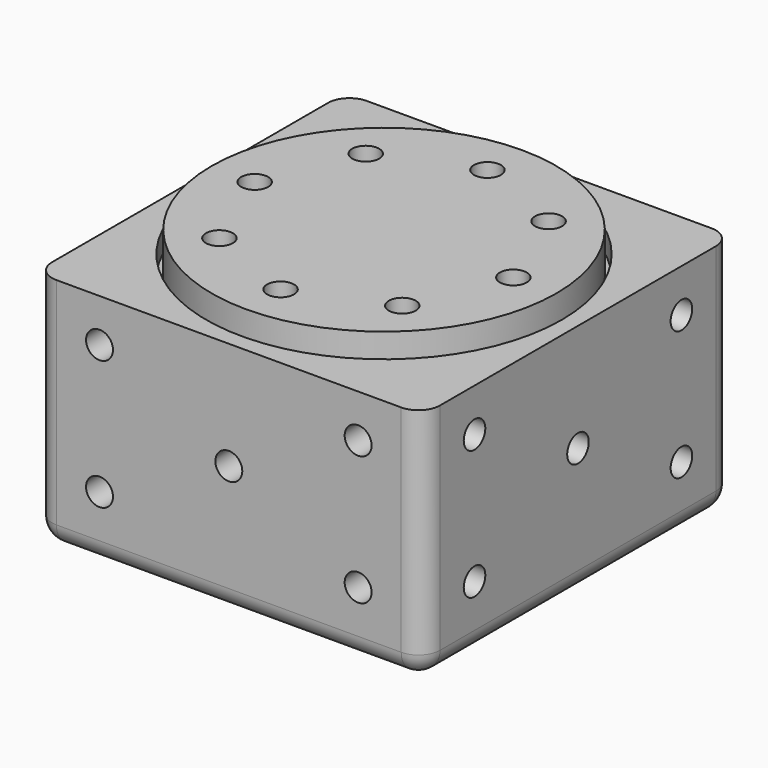
from build123d import *

# Parameters (mm, degrees)
F0_W      = 36
F0_H      = 24
F1_DEPTH  = 18
F5_W      = 36
F5_H      = 36
F5_R      = 16
F6_DEPTH  = 2
F8_R      = 16.5
F8_R_2    = 16
F9_DEPTH  = 2
F10_R     = 2
F2_R      = 1.25
F13_DEPTH = 36.001
F3_R      = 1.25
F14_DEPTH = 36.001
F4_R      = 1.25
F15_DEPTH = 3
F7_R      = 1.25
F16_DEPTH = 3


# Not quite as in the source:
# - a feature of the source that left no trace in its solid (it failed there, or was rolled back) is left out


with BuildPart() as f1:
    # F0 (on Right) → F1 (new body, symmetric)
    with BuildSketch(Plane.YZ):
        Rectangle(F0_W, F0_H)
    extrude(amount=F1_DEPTH, both=True)

    # F5 (on face) → F6 (cut)
    with BuildSketch(Plane.XY.offset(12)):
        Rectangle(F5_W, F5_H)
        Circle(F5_R, mode=Mode.SUBTRACT)
    extrude(amount=-F6_DEPTH, mode=Mode.SUBTRACT)

    # F8 (on face) → F9 (cut)
    with BuildSketch(Plane.XY.offset(10)):
        Circle(F8_R)
        Circle(F8_R_2, mode=Mode.SUBTRACT)
    extrude(amount=-F9_DEPTH, mode=Mode.SUBTRACT)

    # F10
    f10_edges = [f1.edges().sort_by_distance(p)[0] for p in [
        (-18, -18, -1),
        (-18, 18, -1),
        (18, -18, -1),
        (-18, 0, -12),
        (0, 18, -12),
        (18, 0, -12),
        (0, -18, -12),
        (18, 18, -1),
    ]]
    fillet(f10_edges, radius=F10_R)

    # F2 (on face) → F13 (cut, through all)
    with BuildSketch(Plane.XZ.offset(18)):
        with Locations((-12, 6)):
            Circle(F2_R)
        with Locations((12, 6)):
            Circle(F2_R)
        Circle(F2_R)
        with Locations((-12, -6)):
            Circle(F2_R)
        with Locations((12, -6)):
            Circle(F2_R)
    extrude(amount=-F13_DEPTH, mode=Mode.SUBTRACT)

    # F3 (on face) → F14 (cut, through all)
    with BuildSketch(Plane(origin=(-18, 0, 0), x_dir=(0, -1, 0), z_dir=(-1, 0, 0))):
        with Locations((-12, 6)):
            Circle(F3_R)
        with Locations((-12, -6)):
            Circle(F3_R)
        Circle(F3_R)
        with Locations((12, -6)):
            Circle(F3_R)
        with Locations((12, 6)):
            Circle(F3_R)
    extrude(amount=-F14_DEPTH, mode=Mode.SUBTRACT)

    # F4 (on face) → F15 (cut)
    with BuildSketch(Plane.XY.offset(12)):
        with Locations((12, 0)):
            Circle(F4_R)
        with Locations((8.4852813742, 8.4852813742)):
            Circle(F4_R)
        with Locations((0, 12)):
            Circle(F4_R)
        with Locations((-8.4852813742, 8.4852813742)):
            Circle(F4_R)
        with Locations((-12, 0)):
            Circle(F4_R)
        with Locations((-8.4852813742, -8.4852813742)):
            Circle(F4_R)
        with Locations((0, -12)):
            Circle(F4_R)
        with Locations((8.4852813742, -8.4852813742)):
            Circle(F4_R)
    extrude(amount=-F15_DEPTH, mode=Mode.SUBTRACT)

    # F7 (on face) → F16 (cut)
    with BuildSketch(Plane(origin=(0, 0, -12), x_dir=(1, 0, 0), z_dir=(0, 0, -1))):
        with Locations((-12, -12)):
            Circle(F7_R)
        with Locations((-12, 12)):
            Circle(F7_R)
        Circle(F7_R)
        with Locations((12, -12)):
            Circle(F7_R)
        with Locations((12, 12)):
            Circle(F7_R)
    extrude(amount=-F16_DEPTH, mode=Mode.SUBTRACT)


solid = f1.part
